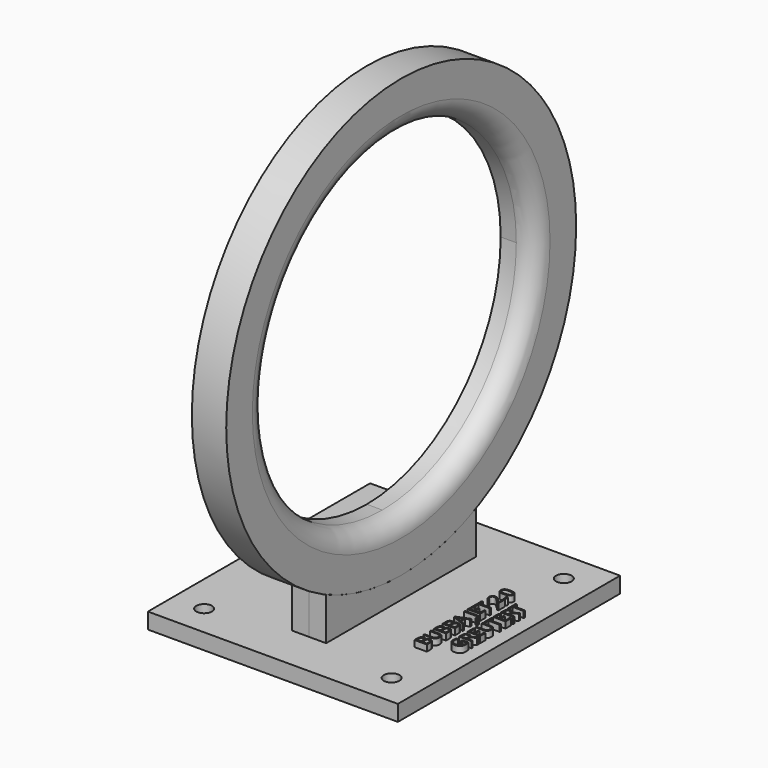
from build123d import *

# Parameters (mm, degrees)
F0_W          = 20
F0_H          = 22.225
F1_DEPTH      = 2.54
F5_DEPTH      = 2.75
F8_DEPTH      = 2.75
F11_R         = 1.25
F12_DEPTH     = 25
F13_TEXT_SIZE = 2.777778
F14_DEPTH     = 1


# Not quite as in the source:
# - a fillet or chamfer that OpenCascade refuses, or shapes differently, is made with other operations: its cross-section is extruded or revolved along the edge and cut away or added
# - Text() gives the source's letters only with a copy of the font that has no kerning and outlines rounded to 1/6400 em; it was checked with that copy


with BuildPart() as f1:
    # F0 (on Top) → F1 (new body)
    with BuildSketch(Plane.XY):
        with Locations((10, 11.1125)):
            Rectangle(F0_W, F0_H)
    extrude(amount=F1_DEPTH)

    # F3: F1 across plane


with BuildPart() as f1_1:
    add(f1.part)
    add(f1.part.mirror(Plane.YZ))

    # F4: F1 across plane


with BuildPart() as f1_2:
    add(f1_1.part)
    add(f1_1.part.mirror(Plane.XZ))


with BuildPart() as f5:
    # F2 (on Right) → F5 (new body)
    with BuildSketch(Plane.YZ):
        with BuildLine():
            ThreePointArc((0, 6), (24.748737, 16.251263), (35, 41))
            ThreePointArc((35, 41), (-24.748737, 65.748737), (0, 6))
        make_face()
        with BuildLine():
            ThreePointArc((26.775, 41), (18.932784, 22.067216), (0, 14.225))
            ThreePointArc((0, 14.225), (-18.932784, 59.932784), (26.775, 41))
        make_face(mode=Mode.SUBTRACT)
    extrude(amount=F5_DEPTH)

    # F6: F5 across plane


with BuildPart() as f5_1:
    add(f5.part)
    add(f5.part.mirror(Plane.YZ))

    # F10: fillet of radius 3 on 1 edges, made by hand

    # F10_s1 → F10_t2 (revolve, cut)
    with BuildSketch(Plane.XY.offset(41)):
        with BuildLine():
            ThreePointArc((2.75, 29.775), (1.87132, 27.65368), (-0.25, 26.775))
            Line((-0.25, 26.775), (2.75, 26.775))
            Line((2.75, 26.775), (2.75, 29.775))
        make_face()
    revolve(axis=Axis((2.75, 0, 41), (1, 0, 0)), mode=Mode.SUBTRACT)


with BuildPart() as f8:
    # F7 (on Right) → F8 (new body)
    with BuildSketch(Plane.YZ):
        with BuildLine():
            Line((-15, 9.377223), (-15, 2.54))
            Line((-15, 2.54), (15, 2.54))
            Line((15, 2.54), (15, 9.377223))
            ThreePointArc((15, 9.377223), (0, 6), (-15, 9.377223))
        make_face()
    extrude(amount=F8_DEPTH)


with BuildPart() as f9_1:
    # F9: instance of F1
    add(f1_2.part.mirror(Plane.YZ))


with BuildPart() as f9_2:
    # F9: instance of F8
    add(f8.part.mirror(Plane.YZ))


with BuildPart() as f12_tool:
    # F11 (on face) → F12 (new body)
    with BuildSketch(Plane.XY.offset(2.54)):
        with Locations((-15, -17.225)):
            Circle(F11_R)
        with Locations((-15, 17.225)):
            Circle(F11_R)
        with Locations((15, -17.225)):
            Circle(F11_R)
        with Locations((15, 17.225)):
            Circle(F11_R)
    extrude(amount=-F12_DEPTH)


with BuildPart() as f1_3:
    add(f1_2.part)

    # F12: cut by f12_tool
    add(f12_tool.part, mode=Mode.SUBTRACT)


with BuildPart() as f9_1_1:
    add(f9_1.part)

    # F12: cut by f12_tool
    add(f12_tool.part, mode=Mode.SUBTRACT)


with BuildPart() as f14:
    # F13 (on face) → F14 (new body)
    with BuildSketch(Plane.XY.offset(2.54)):
        with Locations(Location((14, -9.20204), (0, 0, 90))):
            Text('BUBBA JET 2.0', F13_TEXT_SIZE, font='Open Sans', text_align=(TextAlign.LEFT, TextAlign.BOTTOM))
        with Locations(Location((17.777778, -7.036675), (0, 0, 90))):
            Text('GREUTERT', F13_TEXT_SIZE, font='Open Sans', text_align=(TextAlign.LEFT, TextAlign.BOTTOM))
    extrude(amount=F14_DEPTH)


solid = Compound([f5_1.part, f8.part, f9_2.part, f1_3.part, f9_1_1.part, f14.part])
